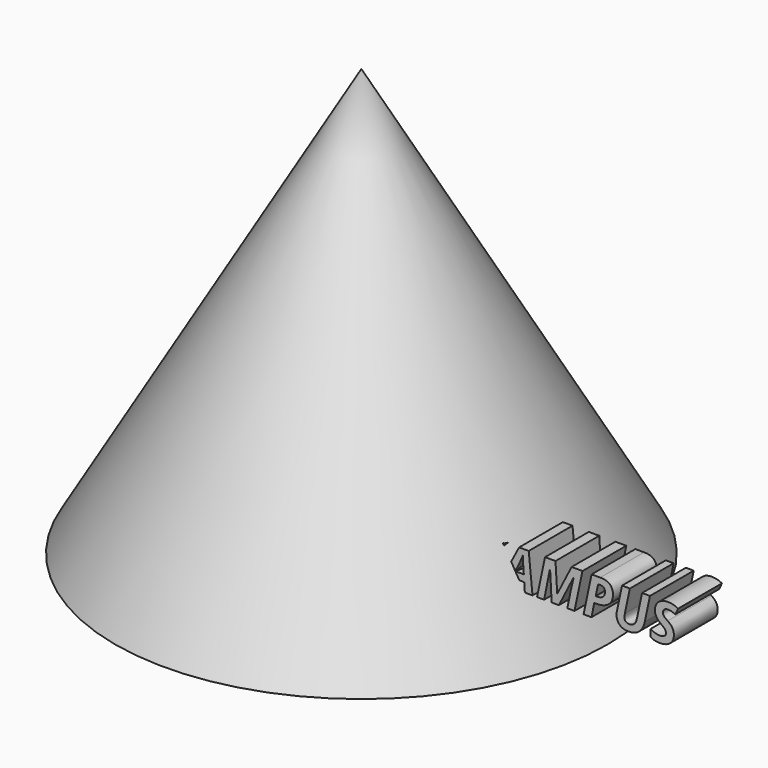
from build123d import *

# Parameters (mm, degrees)
F0_R         = 9
F1_DEPTH     = 16
F1_TAPER     = 30
F2_TEXT_SIZE = 1.9329507702
F3_DEPTH     = 2


# Not quite as in the source:
# - Text() gives the source's letters only with a copy of the font that has no kerning and outlines rounded to 1/6400 em; it was checked with that copy


with BuildPart() as f1:
    # F0 (on Top) → F1 (new body)
    with BuildSketch(Plane.XY):
        Circle(F0_R)
    extrude(amount=F1_DEPTH, taper=F1_TAPER)


with BuildPart() as f3:
    # F2 (on Front) → F3 (new body)
    with BuildSketch(Plane.XZ):
        with Locations((-1.6992390934, 2.0171190992)):
            Text('SALNES CAMPUS', F2_TEXT_SIZE, font='Open Sans', font_style=FontStyle.BOLDITALIC, text_align=(TextAlign.LEFT, TextAlign.BOTTOM))
    extrude(amount=F3_DEPTH)


solid = Compound([f1.part, f3.part])
